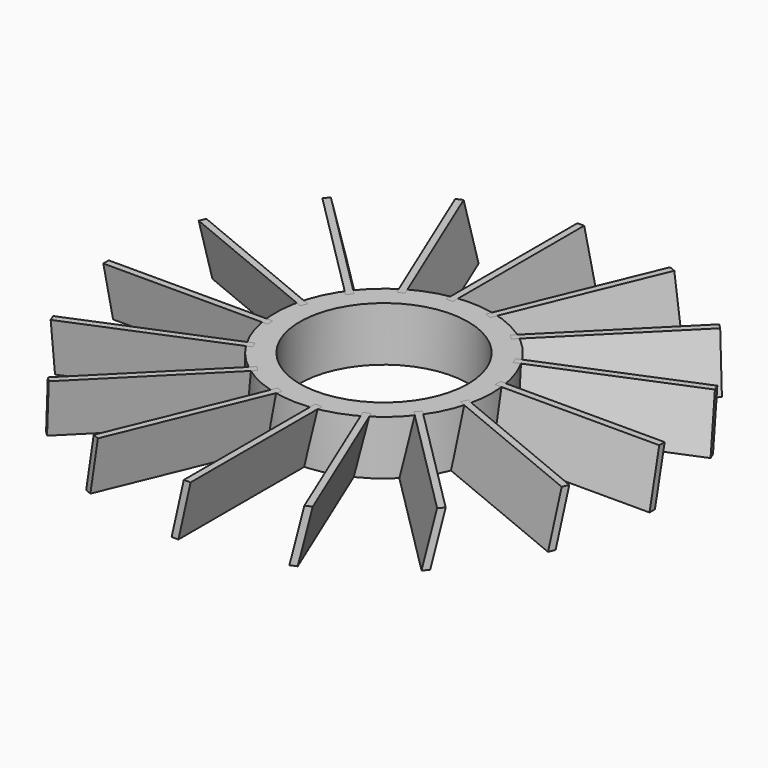
from build123d import *

# Parameters (mm, degrees)
F0_R     = 25.4
F0_R_2   = 19.685
F1_DEPTH = 12.7
F3_START = 23.7242449075
F3_DEPTH = 38.427149877
F4_COUNT = 16


with BuildPart() as f1:
    # F0 (on Top) → F1 (new body)
    with BuildSketch(Plane.XY):
        Circle(F0_R)
        Circle(F0_R_2, mode=Mode.SUBTRACT)
    extrude(amount=F1_DEPTH)


with BuildPart() as f3:
    # F2 (on Front) → F3 (new body)
    with BuildSketch(Plane.XZ.offset(F3_START)):
        Polygon((4.445, 12.7), (2.8575, 12.7), (0, 0), (1.5875, 0), align=None)
    extrude(amount=F3_DEPTH)


with BuildPart() as f4_1:
    # F4: instance of F3
    add(f3.part.rotate(Axis((0, 0, 12.7), (0, 0, 1)), 1 * 360 / F4_COUNT))


with BuildPart() as f4_2:
    # F4: instance of F3
    add(f3.part.rotate(Axis((0, 0, 12.7), (0, 0, 1)), 2 * 360 / F4_COUNT))


with BuildPart() as f4_3:
    # F4: instance of F3
    add(f3.part.rotate(Axis((0, 0, 12.7), (0, 0, 1)), 3 * 360 / F4_COUNT))


with BuildPart() as f4_4:
    # F4: instance of F3
    add(f3.part.rotate(Axis((0, 0, 12.7), (0, 0, 1)), 4 * 360 / F4_COUNT))


with BuildPart() as f4_5:
    # F4: instance of F3
    add(f3.part.rotate(Axis((0, 0, 12.7), (0, 0, 1)), 5 * 360 / F4_COUNT))


with BuildPart() as f4_6:
    # F4: instance of F3
    add(f3.part.rotate(Axis((0, 0, 12.7), (0, 0, 1)), 6 * 360 / F4_COUNT))


with BuildPart() as f4_7:
    # F4: instance of F3
    add(f3.part.rotate(Axis((0, 0, 12.7), (0, 0, 1)), 7 * 360 / F4_COUNT))


with BuildPart() as f4_8:
    # F4: instance of F3
    add(f3.part.rotate(Axis((0, 0, 12.7), (0, 0, 1)), 8 * 360 / F4_COUNT))


with BuildPart() as f4_9:
    # F4: instance of F3
    add(f3.part.rotate(Axis((0, 0, 12.7), (0, 0, 1)), 9 * 360 / F4_COUNT))


with BuildPart() as f4_10:
    # F4: instance of F3
    add(f3.part.rotate(Axis((0, 0, 12.7), (0, 0, 1)), 10 * 360 / F4_COUNT))


with BuildPart() as f4_11:
    # F4: instance of F3
    add(f3.part.rotate(Axis((0, 0, 12.7), (0, 0, 1)), 11 * 360 / F4_COUNT))


with BuildPart() as f4_12:
    # F4: instance of F3
    add(f3.part.rotate(Axis((0, 0, 12.7), (0, 0, 1)), 12 * 360 / F4_COUNT))


with BuildPart() as f4_13:
    # F4: instance of F3
    add(f3.part.rotate(Axis((0, 0, 12.7), (0, 0, 1)), 13 * 360 / F4_COUNT))


with BuildPart() as f4_14:
    # F4: instance of F3
    add(f3.part.rotate(Axis((0, 0, 12.7), (0, 0, 1)), 14 * 360 / F4_COUNT))


with BuildPart() as f4_15:
    # F4: instance of F3
    add(f3.part.rotate(Axis((0, 0, 12.7), (0, 0, 1)), 15 * 360 / F4_COUNT))


solid = Compound([f1.part, f3.part, f4_1.part, f4_2.part, f4_3.part, f4_4.part, f4_5.part, f4_6.part, f4_7.part, f4_8.part, f4_9.part, f4_10.part, f4_11.part, f4_12.part, f4_13.part, f4_14.part, f4_15.part])
